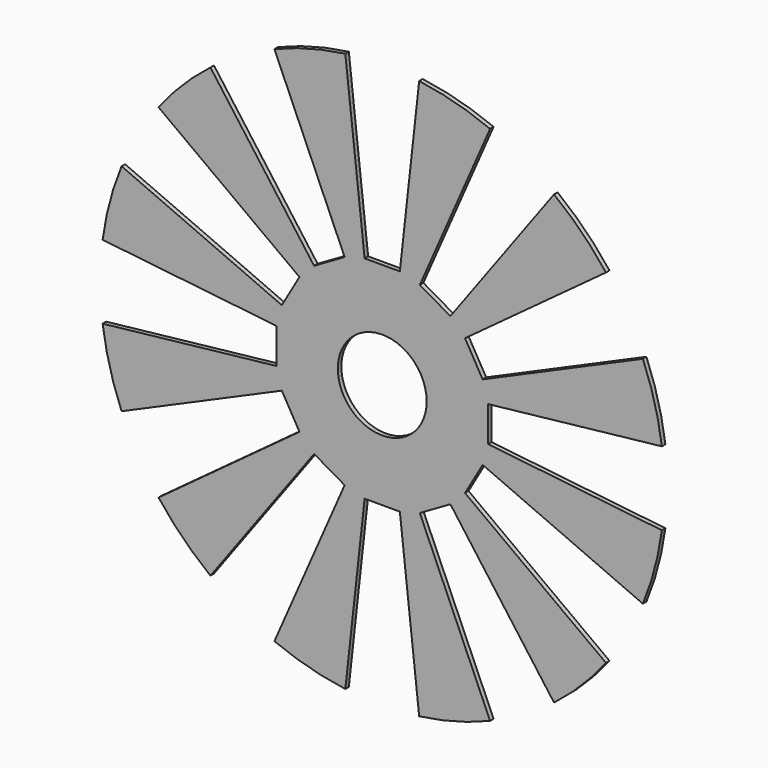
from build123d import *

# Parameters (mm, degrees)
F0_R            = 25.4
F0_R_2          = 4
F1_DEPTH        = 0.1984375
F3_DEPTH        = 25.4
F3_COPIES_COUNT = 12


# Not quite as in the source:
# - a pattern or mirror of a feature is missing from the dataset's text; its kind, count and spacing are read off the source's solid


with BuildPart() as f1:
    # F0 (on Front) → F1 (new body, symmetric)
    with BuildSketch(Plane.XZ):
        Circle(F0_R)
        Circle(F0_R_2, mode=Mode.SUBTRACT)
    extrude(amount=F1_DEPTH, both=True)

    # F2 (on face) → F3 (cut)
    with BuildSketch(Plane.XZ.offset(0.1984375)):
        Polygon((-1.5875, 9.525), (1.5875, 9.525), (3.3247541667, 25.1814616282), (0, 29.9078127353), (-3.3247541667, 25.1814616282), align=None)
    f3 = extrude(amount=-F3_DEPTH, mode=Mode.SUBTRACT)

    # F3_copies: F3 ×12 about axis
    f3_copies_axis = Axis((0, 0, 0), (0, 1, 0))
    for i in range(1, F3_COPIES_COUNT):
        add(f3.rotate(f3_copies_axis, i * 360 / F3_COPIES_COUNT), mode=Mode.SUBTRACT)


solid = f1.part
